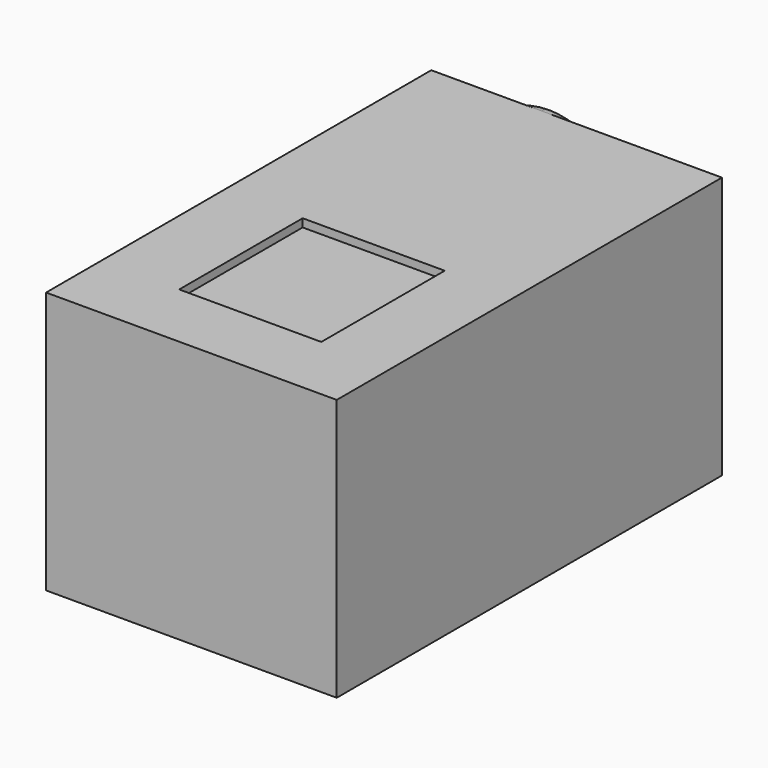
from build123d import *

# Parameters (mm, degrees)
F0_W     = 35.8
F0_H     = 59.3
F1_DEPTH = 32.3
F2_W     = 17.5
F2_H     = 19
F3_DEPTH = 1
F5_DEPTH = 2
F6_R     = 1.99999
F7_DEPTH = 1


# Not quite as in the source:
# - a fillet or chamfer is up to 0.001 mm smaller than in the source, because OpenCascade refuses the exact size


with BuildPart() as f1:
    # F0 (on Top) → F1 (new body)
    with BuildSketch(Plane.XY):
        Rectangle(F0_W, F0_H)
    extrude(amount=F1_DEPTH)

    # F2 (on face) → F3 (cut)
    with BuildSketch(Plane.XY.offset(32.3)):
        with Locations((0.45, -11.65)):
            Rectangle(F2_W, F2_H)
    extrude(amount=-F3_DEPTH, mode=Mode.SUBTRACT)

    # F4 (on face) → F5 (join)
    with BuildSketch(Plane(origin=(0, 29.65, 0), x_dir=(-1, 0, 0), z_dir=(0, 1, 0))):
        with BuildLine():
            ThreePointArc((4.3000000252, 32.3), (-1.9932503615, 17.1067496563), (13.2, 23.4))
            ThreePointArc((13.2, 23.4), (10.5932503615, 29.6932503437), (4.3000000252, 32.3))
        make_face()
    extrude(amount=F5_DEPTH)

    # F6 (radius 2 in the source; OpenCascade refuses exactly that, so slightly less here)
    f6_edges = [f1.edges().sort_by_distance(p)[0] for p in [
        (4.6, 31.65, 23.4),
    ]]
    fillet(f6_edges, radius=F6_R)

    # F7 (cut): a face of the model
    f7_faces = [f1.faces().sort_by_distance(p)[0] for p in [
        (-4.3, 31.65, 23.4),
    ]]
    extrude(f7_faces, amount=-F7_DEPTH, mode=Mode.SUBTRACT)


solid = f1.part
